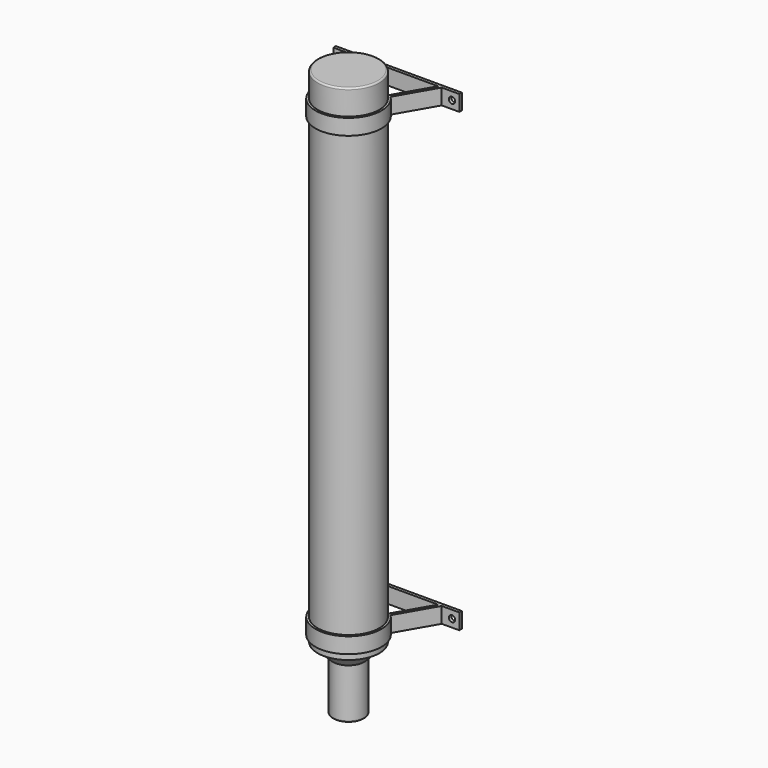
from build123d import *

# Parameters (mm, degrees)
F0_R      = 98
F1_DEPTH  = 900
F2_R      = 98
F2_R_2    = 50
F3_DEPTH  = 200
F4_SIZE   = 40
F5_R      = 5
F8_DEPTH  = 50
F9_R      = 6.75
F9_R_2    = 10
F10_DEPTH = 10.001


# Not quite as in the source:
# - a pattern or mirror of a feature is missing from the dataset's text; its kind, count and spacing are read off the source's solid


with BuildPart() as f1:
    # F0 (on Top) → F1 (new body, symmetric)
    with BuildSketch(Plane.XY):
        Circle(F0_R)
    extrude(amount=F1_DEPTH, both=True)

    # F2 (on face) → F3 (cut)
    with BuildSketch(Plane(origin=(0, 0, -900), x_dir=(1, 0, 0), z_dir=(0, 0, -1))):
        Circle(F2_R)
        Circle(F2_R_2, mode=Mode.SUBTRACT)
    extrude(amount=-F3_DEPTH, mode=Mode.SUBTRACT)

    # F4
    f4_edges = [f1.edges().sort_by_distance(p)[0] for p in [
        (-50, 0, -700),
    ]]
    chamfer(f4_edges, length=F4_SIZE)

    # F5
    f5_edges = [f1.edges().sort_by_distance(p)[0] for p in [
        (-50, 0, -900),
        (-98, 0, 900),
    ]]
    fillet(f5_edges, radius=F5_R)

    # F7 (on offset) → F8 (join)
    with BuildSketch(Plane(origin=(0, 0, -680), x_dir=(1, 0, 0), z_dir=(0, 0, -1))):
        Polygon((76.2233031652, -72.2150126676), (65.2159465136, -73.14971169), (132.6794919243, -190), (-132.6794919243, -190), (-65.2159465136, -73.14971169), (-76.2233031652, -72.2150126676), (-144.2264973081, -190), (-200, -190), (-200, -200), (-150, -200), (150, -200), (200, -200), (200, -190), (144.2264973081, -190), align=None)
        with BuildLine():
            ThreePointArc((-65.2159465136, -73.14971169), (0, 98), (65.2159465136, -73.14971169))
            Line((65.2159465136, -73.14971169), (76.2233031652, -72.2150126676))
            ThreePointArc((76.2233031652, -72.2150126676), (0, 105), (-76.2233031652, -72.2150126676))
            Line((-76.2233031652, -72.2150126676), (-65.2159465136, -73.14971169))
        make_face()
    f8 = extrude(amount=-F8_DEPTH)

    # F8_copies: F8 across plane
    add(f8.mirror(Plane.XY.offset(70)))

    # F9 (on face) → F10 (cut, through all)
    with BuildSketch(Plane.XZ.offset(-190)):
        with Locations((-172.1132486541, -655)):
            Circle(F9_R)
        with Locations((176.858574152, -655)):
            Circle(F9_R_2)
    f10 = extrude(amount=-F10_DEPTH, mode=Mode.SUBTRACT)

    # F10_copies: F10 across plane
    add(f10.mirror(Plane.XY.offset(70)), mode=Mode.SUBTRACT)


solid = f1.part
